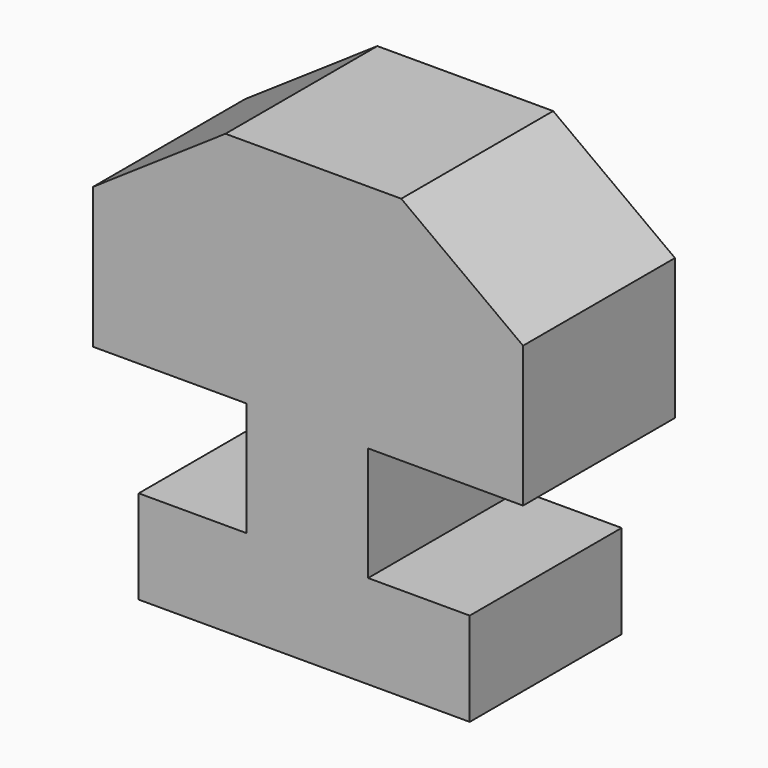
from build123d import *

# Parameters (mm, degrees)
F0_W     = 16.2341720425
F0_H     = 15.2690820396
F1_DEPTH = 25.4
F2_DEPTH = 25.4


# Not quite as in the source:
# - a feature names something its author has since deleted; it is built from what else it names


with BuildPart() as f1:
    # F0 (on Front) → F1 (new body)
    with BuildSketch(Plane.XZ):
        Polygon((-9.2177884653, -27.9424227774), (7.0163835771, -27.9424227774), (27.7444086969, -27.9424227774), (27.7444086969, -9.1097736731), (11.4521000938, 2.9011261649), (-12.0625765994, 2.9011261649), (-29.7747123986, -9.1097736731), (-29.7747123986, -27.9424227774), align=None)
        with Locations((-1.1007024441, -35.5769637972)):
            Rectangle(F0_W, F0_H)
    extrude(amount=F1_DEPTH)

    # F0 (on Front) → F2 (join)
    with BuildSketch(Plane.XZ):
        Polygon((-23.6670821905, -55.7321608067), (20.6132540479, -55.7321608067), (20.6132540479, -43.211504817), (7.0163835771, -43.211504817), (-9.2177884653, -43.211504817), (-23.6670821905, -43.211504817), align=None)
    extrude(amount=F2_DEPTH)


solid = f1.part
